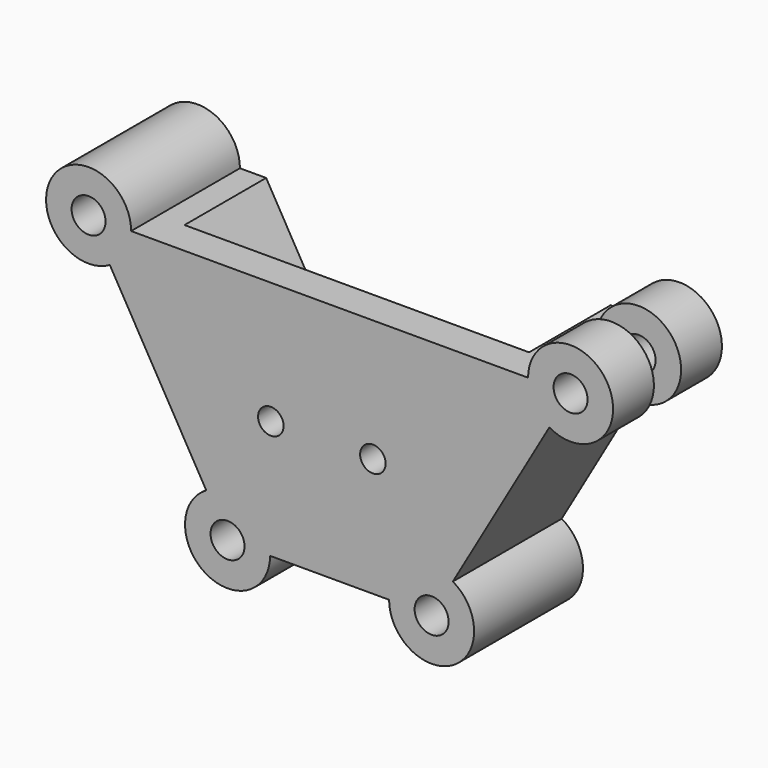
from build123d import *

# Parameters (mm, degrees)
F0_R     = 12.7
F1_DEPTH = 50.8
F3_DEPTH = 76.2
F4_R     = 38.1
F5_DEPTH = 12.7
F6_R     = 9.525
F7_DEPTH = 42.418


# Not quite as in the source:
# - the program builds the solid bodies; features that only make, move or delete a surface that nothing else refers to are left out


with BuildPart() as f1:
    # F0 (on Front) → F1 (new body, symmetric)
    with BuildSketch(Plane.XZ):
        with BuildLine():
            Line((154.00903388, 91.1349219612), (-142.45976612, 91.1349219612))
            ThreePointArc((-142.45976612, 91.1349219612), (-201.7060726901, 107.0099219612), (-158.33476612, 63.638615391))
            Line((-158.33476612, 63.638615391), (-86.30036612, -61.1286253017))
            ThreePointArc((-86.30036612, -61.1286253017), (-86.30036612, -116.121238442), (-38.67536612, -88.6249318719))
            Line((-38.67536612, -88.6249318719), (50.22463388, -88.6249318719))
            ThreePointArc((50.22463388, -88.6249318719), (97.84963388, -116.121238442), (97.84963388, -61.1286253017))
            Line((97.84963388, -61.1286253017), (169.88403388, 63.638615391))
            ThreePointArc((169.88403388, 63.638615391), (213.2553404502, 107.0099219612), (154.00903388, 91.1349219612))
        make_face()
        with Locations((-70.42536612, -88.6249318719)):
            Circle(F0_R, mode=Mode.SUBTRACT)
        with Locations((81.97463388, -88.6249318719)):
            Circle(F0_R, mode=Mode.SUBTRACT)
        with Locations((-174.20976612, 91.1349219612)):
            Circle(F0_R, mode=Mode.SUBTRACT)
        with Locations((185.75903388, 91.1349219612)):
            Circle(F0_R, mode=Mode.SUBTRACT)
    extrude(amount=-F1_DEPTH, both=True)

    # F2 (on face) → F3 (cut)
    with BuildSketch(Plane(origin=(0, 50.8, 0), x_dir=(-1, 0, 0), z_dir=(0, 1, 0))):
        Polygon((122.883327189, 91.1349219612), (-134.4325949491, 91.1349219612), (-58.2325949491, -40.8473495756), (46.683327189, -40.8473495756), align=None)
    extrude(amount=-F3_DEPTH, mode=Mode.SUBTRACT)

    # F4 (on Front) → F5 (cut, symmetric)
    with BuildSketch(Plane.XZ):
        with Locations((186.0332787037, 91.5846452117)):
            Circle(F4_R)
    extrude(amount=F5_DEPTH, both=True, mode=Mode.SUBTRACT)

    # F6 (on face) → F7 (cut, symmetric)
    with BuildSketch(Plane(origin=(0, -25.4, 0), x_dir=(-1, 0, 0), z_dir=(0, 1, 0))):
        with BuildLine():
            ThreePointArc((47.625, 0), (38.1, 9.525), (28.575, 0))
            ThreePointArc((28.575, 0), (38.1, -9.525), (47.625, 0))
        make_face()
        with Locations((-38.1, 0)):
            Circle(F6_R)
    extrude(amount=F7_DEPTH, both=True, mode=Mode.SUBTRACT)


solid = f1.part
